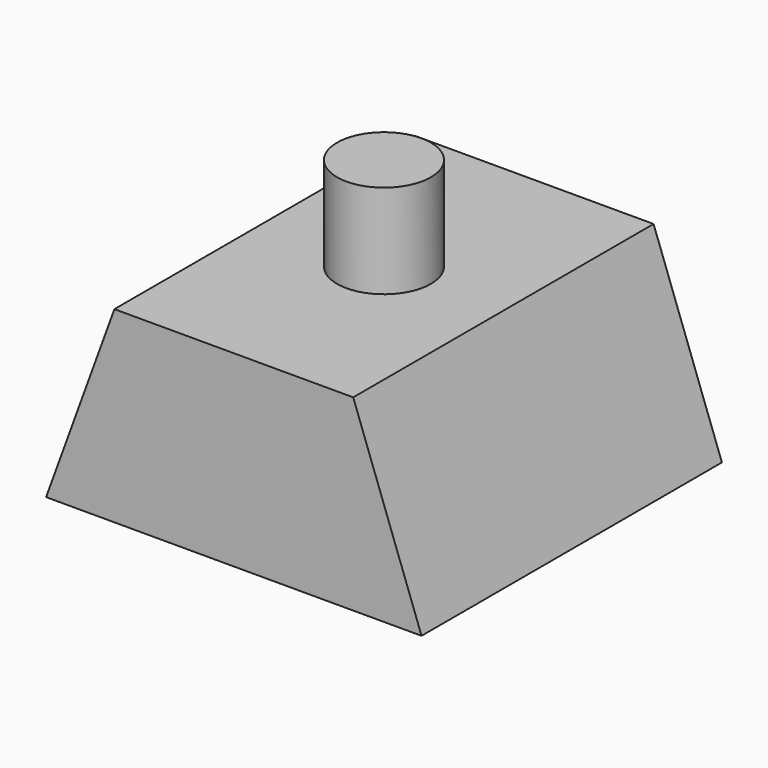
from build123d import *

# Parameters (mm, degrees)
F1_DEPTH = 20
F2_R     = 2.5
F3_DEPTH = 5


# Not quite as in the source:
# - a feature names something its author has since deleted; it is built from what else it names


with BuildPart() as f1:
    # F0 (on Front) → F1 (new body)
    with BuildSketch(Plane.XZ):
        Polygon((-20, 0), (0, 0), (-3.64, 10), (-16.36, 10), align=None)
    extrude(amount=F1_DEPTH)

    # F2 (on face) → F3 (join)
    with BuildSketch(Plane.XY.offset(10)):
        with Locations((-10, -10)):
            Circle(F2_R)
    extrude(amount=F3_DEPTH)


solid = f1.part
